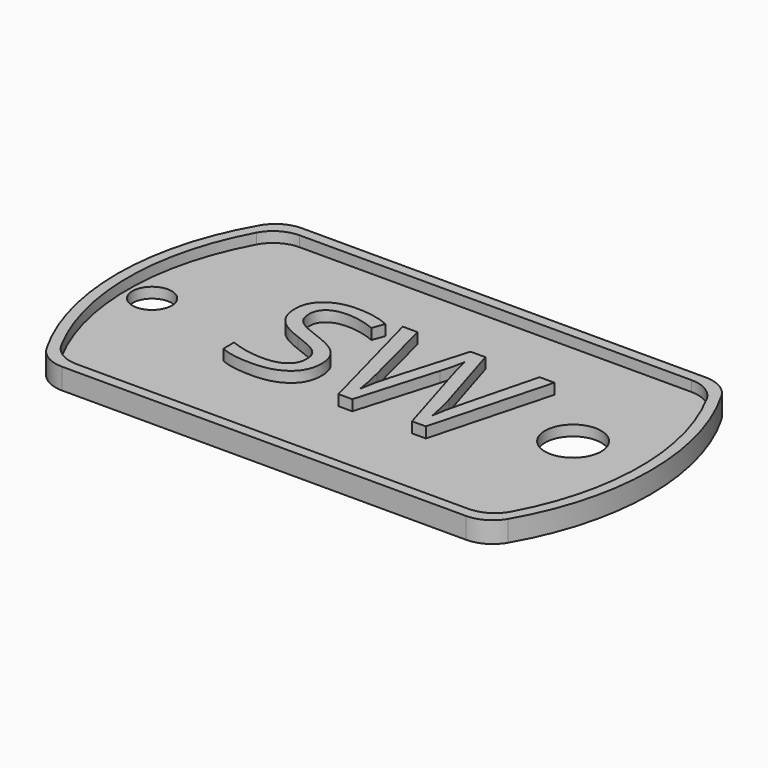
from build123d import *

# Parameters (mm, degrees)
F0_R         = 1.8739594118
F1_DEPTH     = 1
F3_DEPTH     = 1
F4_TEXT_SIZE = 16.0777378672
F5_DEPTH     = 1.016
F6_R         = 2.6794079617
F7_DEPTH     = 2.54


# Not quite as in the source:
# - Text() gives the source's letters only with a copy of the font that has no kerning and outlines rounded to 1/6400 em; it was checked with that copy


with BuildPart() as f1:
    # F0 (on Top) → F1 (new body)
    with BuildSketch(Plane.XY):
        with BuildLine():
            ThreePointArc((-19.2474145991, 14.2875), (-20.8349145991, 13.862130657), (-21.9970452561, 12.7))
            ThreePointArc((-21.9970452561, 12.7), (-25.4, 0), (-21.9970452561, -12.7))
            ThreePointArc((-21.9970452561, -12.7), (-20.8349145991, -13.862130657), (-19.2474145991, -14.2875))
            Line((-19.2474145991, -14.2875), (19.2474145991, -14.2875))
            ThreePointArc((19.2474145991, -14.2875), (20.8349145991, -13.862130657), (21.9970452561, -12.7))
            ThreePointArc((21.9970452561, -12.7), (25.4, 0), (21.9970452561, 12.7))
            ThreePointArc((21.9970452561, 12.7), (20.8349145991, 13.862130657), (19.2474145991, 14.2875))
            Line((19.2474145991, 14.2875), (-19.2474145991, 14.2875))
        make_face()
        with Locations((-22.0978986472, 0)):
            Circle(F0_R, mode=Mode.SUBTRACT)
    extrude(amount=F1_DEPTH)

    # F2 (on face) → F3 (join)
    with BuildSketch(Plane.XY.offset(1)):
        with BuildLine():
            Line((19.2474145991, 14.2875), (-19.2474145991, 14.2875))
            ThreePointArc((-19.2474145991, 14.2875), (-20.8349145991, 13.862130657), (-21.9970452561, 12.7))
            ThreePointArc((-21.9970452561, 12.7), (-25.4, 0), (-21.9970452561, -12.7))
            ThreePointArc((-21.9970452561, -12.7), (-20.8349145991, -13.862130657), (-19.2474145991, -14.2875))
            Line((-19.2474145991, -14.2875), (19.2474145991, -14.2875))
            ThreePointArc((19.2474145991, -14.2875), (20.8349145991, -13.862130657), (21.9970452561, -12.7))
            ThreePointArc((21.9970452561, -12.7), (25.4, 0), (21.9970452561, 12.7))
            ThreePointArc((21.9970452561, 12.7), (20.8349145991, 13.862130657), (19.2474145991, 14.2875))
        make_face()
        with BuildLine():
            ThreePointArc((-21.4526124879, 11.6252061249), (-20.2856017842, 12.8404540819), (-18.6611352482, 13.2875))
            Line((-18.6611352482, 13.2875), (18.6611352482, 13.2875))
            ThreePointArc((18.6611352482, 13.2875), (20.2856017842, 12.8404540819), (21.4526124879, 11.6252061249))
            ThreePointArc((21.4526124879, 11.6252061249), (24.4, 0), (21.4526124879, -11.6252061249))
            ThreePointArc((21.4526124879, -11.6252061249), (20.2856017842, -12.8404540819), (18.6611352482, -13.2875))
            Line((18.6611352482, -13.2875), (-18.6611352482, -13.2875))
            ThreePointArc((-18.6611352482, -13.2875), (-20.2856017842, -12.8404540819), (-21.4526124879, -11.6252061249))
            ThreePointArc((-21.4526124879, -11.6252061249), (-24.4, 0), (-21.4526124879, 11.6252061249))
        make_face(mode=Mode.SUBTRACT)
    extrude(amount=F3_DEPTH)

    # F4 (on face) → F5 (join)
    with BuildSketch(Plane.XY.offset(1)):
        with Locations((-12.5048193149, -4.9125263467)):
            Text('SW', F4_TEXT_SIZE, font='Open Sans', text_align=(TextAlign.LEFT, TextAlign.BOTTOM))
    extrude(amount=F5_DEPTH)

    # F6 (on face) → F7 (cut)
    with BuildSketch(Plane.XY.offset(1)):
        with Locations((16.7385805398, 1.6000774922)):
            Circle(F6_R)
    extrude(amount=-F7_DEPTH, mode=Mode.SUBTRACT)


solid = f1.part
